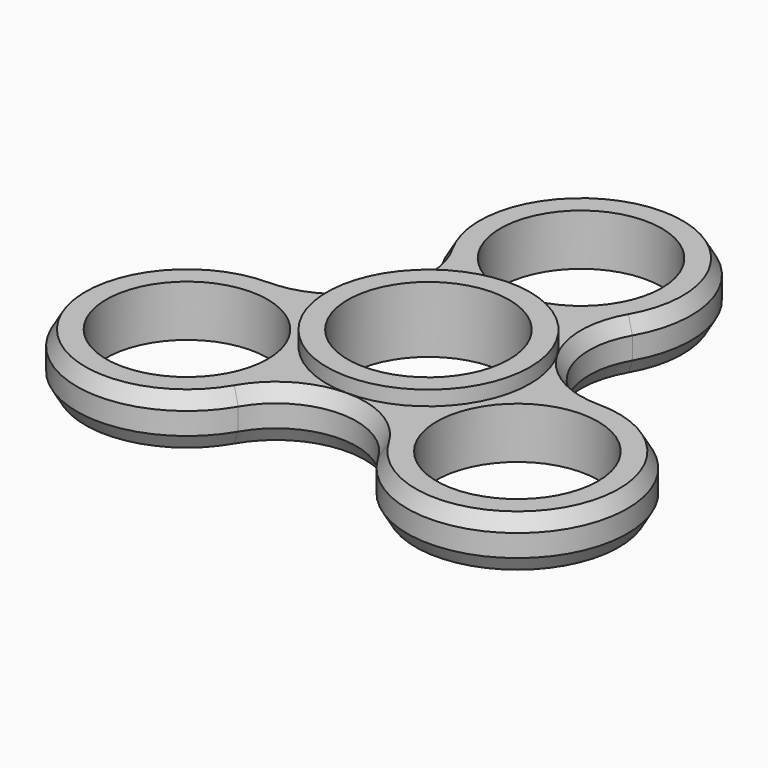
from build123d import *

# Parameters (mm, degrees)
F0_R          = 11
F1_DEPTH      = 3.5
F2_R          = 11
F3_DEPTH      = 3.501
F3_DEPTH_BACK = 3.501
F4_T2_ANGLE   = 240
F4_T4_ANGLE   = 240
F4_T6_ANGLE   = 120
F4_T8_ANGLE   = 120
F4_T10_ANGLE  = 240
F4_T12_ANGLE  = 240
F4_T14_ANGLE  = 120
F4_T16_ANGLE  = 120
F4_T18_ANGLE  = 240
F4_T20_ANGLE  = 240
F4_T22_ANGLE  = 120
F4_T24_ANGLE  = 120
F5_R          = 13.8452994616
F5_R_2        = 11
F6_DEPTH      = 2


# Not quite as in the source:
# - a fillet or chamfer that OpenCascade refuses, or shapes differently, is made with other operations: its cross-section is extruded or revolved along the edge and cut away or added


with BuildPart() as f1:
    # F0 (on Top) → F1 (new body, symmetric)
    with BuildSketch(Plane.XY):
        with BuildLine():
            ThreePointArc((-22.5166604984, 2), (-35.5070415552, -20.5), (-9.5262794416, -20.5))
            ThreePointArc((-9.5262794416, -20.5), (0, -15), (9.5262794416, -20.5))
            ThreePointArc((9.5262794416, -20.5), (35.5070415552, -20.5), (22.5166604984, 2))
            ThreePointArc((22.5166604984, 2), (12.9903810568, 7.5), (12.9903810568, 18.5))
            ThreePointArc((12.9903810568, 18.5), (0, 41), (-12.9903810568, 18.5))
            ThreePointArc((-12.9903810568, 18.5), (-12.9903810568, 7.5), (-22.5166604984, 2))
        make_face()
        with Locations((-22.5166604984, -13)):
            Circle(F0_R, mode=Mode.SUBTRACT)
        with Locations((22.5166604984, -13)):
            Circle(F0_R, mode=Mode.SUBTRACT)
        Circle(F0_R, mode=Mode.SUBTRACT)
        with Locations((0, 26)):
            Circle(F0_R, mode=Mode.SUBTRACT)
    extrude(amount=F1_DEPTH, both=True)

    # F2 (on Top) → F3 (cut, two sides)
    with BuildSketch(Plane.XY) as f3_sk:
        Circle(F2_R)
    extrude(amount=-F3_DEPTH, mode=Mode.SUBTRACT)
    extrude(f3_sk.sketch, amount=F3_DEPTH_BACK, mode=Mode.SUBTRACT)

    # F4: chamfer of 2 x 1.1547005384 on 12 edges, made by hand

    # F4_s1 → F4_t2 (revolve, cut)
    with BuildSketch(Plane.YZ.offset(-22.5166604984)):
        Polygon((0.8452994616, 3.5), (2, 1.5), (2, 3.5), align=None)
    revolve(axis=Axis((-22.5166604984, -13, 3.5), (0, 0, 1)), revolution_arc=F4_T2_ANGLE, mode=Mode.SUBTRACT)

    # F4_s3 → F4_t4 (revolve, cut)
    with BuildSketch(Plane.YZ.offset(-22.5166604984)):
        Polygon((2, -1.5), (0.8452994616, -3.5), (2, -3.5), align=None)
    revolve(axis=Axis((-22.5166604984, -13, -3.5), (0, 0, 1)), revolution_arc=F4_T4_ANGLE, mode=Mode.SUBTRACT)

    # F4_s5 → F4_t6 (revolve, cut)
    with BuildSketch(Plane(origin=(-11.2583302492, 19.5, 0), x_dir=(0, 0, 1), z_dir=(-0.5, 0.8660254038, 0))):
        Polygon((-1.5, -2), (-3.5, -0.8452994616), (-3.5, -2), align=None)
    revolve(axis=Axis((-22.5166604984, 13, -3.5), (0, 0, -1)), revolution_arc=F4_T6_ANGLE, mode=Mode.SUBTRACT)

    # F4_s7 → F4_t8 (revolve, cut)
    with BuildSketch(Plane(origin=(-11.2583302492, 19.5, 0), x_dir=(0, 0, 1), z_dir=(-0.5, 0.8660254038, 0))):
        Polygon((1.5, -2), (3.5, -0.8452994616), (3.5, -2), align=None)
    revolve(axis=Axis((-22.5166604984, 13, 3.5), (0, 0, -1)), revolution_arc=F4_T8_ANGLE, mode=Mode.SUBTRACT)

    # F4_s9 → F4_t10 (revolve, cut)
    with BuildSketch(Plane(origin=(11.2583302492, 19.5, 0), x_dir=(0, 0, 1), z_dir=(-0.5, -0.8660254038, 0))):
        Polygon((-1.5, -2), (-3.5, -0.8452994616), (-3.5, -2), align=None)
    revolve(axis=Axis((0, 26, -3.5), (0, 0, 1)), revolution_arc=F4_T10_ANGLE, mode=Mode.SUBTRACT)

    # F4_s11 → F4_t12 (revolve, cut)
    with BuildSketch(Plane(origin=(11.2583302492, 19.5, 0), x_dir=(0, 0, 1), z_dir=(-0.5, -0.8660254038, 0))):
        Polygon((1.5, -2), (3.5, -0.8452994616), (3.5, -2), align=None)
    revolve(axis=Axis((0, 26, 3.5), (0, 0, 1)), revolution_arc=F4_T12_ANGLE, mode=Mode.SUBTRACT)

    # F4_s13 → F4_t14 (revolve, cut)
    with BuildSketch(Plane.YZ.offset(22.5166604984)):
        Polygon((2, -1.5), (0.8452994616, -3.5), (2, -3.5), align=None)
    revolve(axis=Axis((22.5166604984, 13, -3.5), (0, 0, -1)), revolution_arc=F4_T14_ANGLE, mode=Mode.SUBTRACT)

    # F4_s15 → F4_t16 (revolve, cut)
    with BuildSketch(Plane.YZ.offset(22.5166604984)):
        Polygon((2, 1.5), (0.8452994616, 3.5), (2, 3.5), align=None)
    revolve(axis=Axis((22.5166604984, 13, 3.5), (0, 0, -1)), revolution_arc=F4_T16_ANGLE, mode=Mode.SUBTRACT)

    # F4_s17 → F4_t18 (revolve, cut)
    with BuildSketch(Plane(origin=(11.2583302492, -19.5, 0), x_dir=(0, 0, 1), z_dir=(-0.5, 0.8660254038, 0))):
        Polygon((-1.5, -2), (-3.5, -0.8452994616), (-3.5, -2), align=None)
    revolve(axis=Axis((22.5166604984, -13, -3.5), (0, 0, 1)), revolution_arc=F4_T18_ANGLE, mode=Mode.SUBTRACT)

    # F4_s19 → F4_t20 (revolve, cut)
    with BuildSketch(Plane(origin=(11.2583302492, -19.5, 0), x_dir=(0, 0, 1), z_dir=(-0.5, 0.8660254038, 0))):
        Polygon((1.5, -2), (3.5, -0.8452994616), (3.5, -2), align=None)
    revolve(axis=Axis((22.5166604984, -13, 3.5), (0, 0, 1)), revolution_arc=F4_T20_ANGLE, mode=Mode.SUBTRACT)

    # F4_s21 → F4_t22 (revolve, cut)
    with BuildSketch(Plane(origin=(-11.2583302492, -19.5, 0), x_dir=(0, 0, 1), z_dir=(-0.5, -0.8660254038, 0))):
        Polygon((-1.5, -2), (-3.5, -0.8452994616), (-3.5, -2), align=None)
    revolve(axis=Axis((0, -26, -3.5), (0, 0, -1)), revolution_arc=F4_T22_ANGLE, mode=Mode.SUBTRACT)

    # F4_s23 → F4_t24 (revolve, cut)
    with BuildSketch(Plane(origin=(-11.2583302492, -19.5, 0), x_dir=(0, 0, 1), z_dir=(-0.5, -0.8660254038, 0))):
        Polygon((1.5, -2), (3.5, -0.8452994616), (3.5, -2), align=None)
    revolve(axis=Axis((0, -26, 3.5), (0, 0, -1)), revolution_arc=F4_T24_ANGLE, mode=Mode.SUBTRACT)

    # F5 (on face) → F6 (join)
    with BuildSketch(Plane.XY.offset(3.5)):
        Circle(F5_R)
        Circle(F5_R_2, mode=Mode.SUBTRACT)
    extrude(amount=F6_DEPTH)


solid = f1.part
